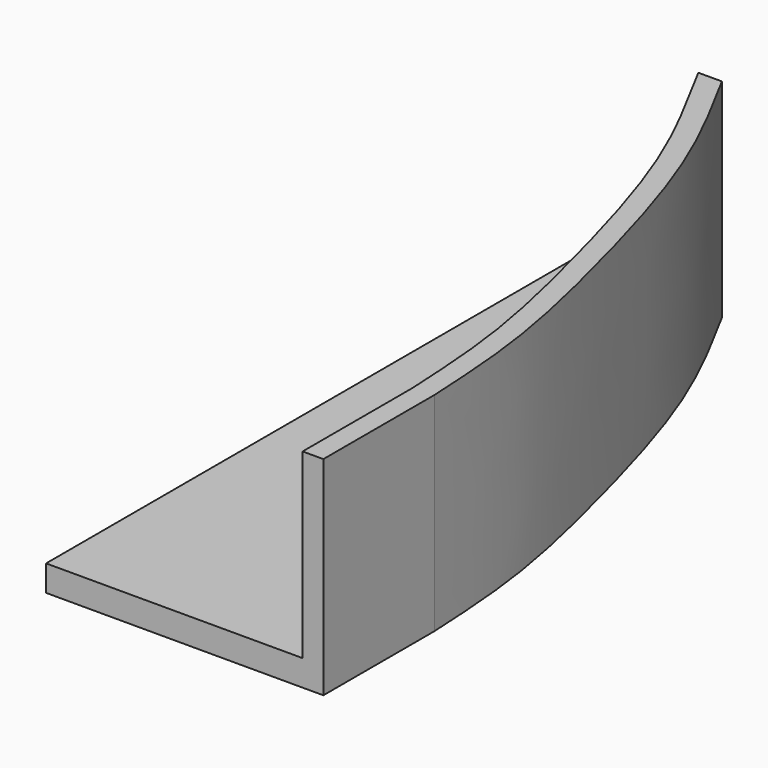
from build123d import *

# Parameters (mm, degrees)
F1_DEPTH = 60
F2_DEPTH = 7.5


# Not quite as in the source:
# - the dataset's text gives a spline's control points without its knots; the knots are read off the source's solid


with BuildPart() as f1:
    # F0 (on Top) → F1 (new body)
    with BuildSketch(Plane.XY):
        with BuildLine():
            Line((-3.4322376549, 127.3491138778), (-10.2491527796, 127.3491138778))
            Line((-10.2491527796, 127.3491138778), (-8.701252002, 124.4790114736))
            add(Edge.make_bspline(
                [(-8.701252002, 124.4790114736), (-7.1362237136, 121.6058887261), (-4.800992375, 117.3185625984), (-1.747416122, 111.541576422), (0.5046891705, 107.1516705554), (2.7109302282, 102.6774335337), (4.5050186798, 98.8556741617), (5.9099551663, 95.7283837822), (6.947576742, 93.3444650289), (7.7980975394, 91.3228569804), (8.4695499974, 89.6828524521), (9.1348820035, 88.0269081744), (9.957166215, 85.9221359954), (11.251973665, 82.4881889813), (12.831222258, 78.0823686514), (14.662666653, 72.6512882748), (16.4302898701, 67.1126017724), (18.134279165, 61.5024770299), (19.7751169491, 55.8567117619), (21.0904401972, 51.1517886054), (22.1119013069, 47.4054001661), (22.8627437246, 44.6087322937), (23.5983740983, 41.8296630381), (24.5595560319, 38.152939528), (25.7198359711, 33.6303684872), (27.0381614496, 28.3164099437), (28.2747953137, 23.1133958726), (29.4220535656, 18.0186567898), (30.4723828119, 13.0297011115), (31.2606871801, 8.9582973415), (31.8355062448, 5.7515670621), (32.2378190146, 3.3713838737), (32.5483276312, 1.4084100397), (32.7814771963, -0.1499496395), (33.0042095884, -1.6999194073), (33.2639776094, -3.6272829064), (33.5480887505, -5.9256145197), (33.806687748, -8.2111304942), (34.1203062464, -11.2436070922), (34.4591587016, -15.0104238238), (34.7976724691, -19.5054666923), (35.1809644079, -25.4820365724), (35.4176012213, -29.9639189701), (35.5761012306, -32.9671092858)],
                knots=[0, 0, 0, 0, 0.0625, 0.09375, 0.125, 0.15625, 0.1875, 0.203125, 0.21875, 0.234375, 0.2421875, 0.25, 0.265625, 0.28125, 0.3125, 0.34375, 0.375, 0.40625, 0.4375, 0.46875, 0.484375, 0.5, 0.515625, 0.53125, 0.5625, 0.59375, 0.625, 0.65625, 0.6875, 0.71875, 0.734375, 0.75, 0.765625, 0.7734375, 0.78125, 0.796875, 0.8125, 0.828125, 0.84375, 0.875, 0.90625, 0.9375, 1, 1, 1, 1], degree=3))
            Line((35.5761012306, -32.9671092858), (35.5761012306, -72.6508861222))
            Line((35.5761012306, -72.6508861222), (41.5677623451, -72.6508861222))
            Line((41.5677623451, -72.6508861222), (41.5677623451, -32.6508861222))
            add(Edge.make_bspline(
                [(-3.4322376549, 127.3491138778), (2.7057866735, 116.0807569713), (15.8535559025, 91.943714127), (30.1753131948, 41.9800249332), (39.8006878737, 0.8308844005), (41.0051328293, -21.9904229426), (41.5677623451, -32.6508861222)],
                knots=[0, 0, 0, 0, 0.2451243363, 0.5250611653, 0.7781429484, 1, 1, 1, 1], degree=3))
        make_face()
    extrude(amount=F1_DEPTH)

    # F0 (on Top) → F2 (join)
    with BuildSketch(Plane.XY):
        with BuildLine():
            Line((-10.2491527796, 127.3491138778), (-38.4322376549, 127.3491138778))
            Line((-38.4322376549, 127.3491138778), (-38.4322376549, -72.6508861222))
            Line((-38.4322376549, -72.6508861222), (35.5761012306, -72.6508861222))
            Line((35.5761012306, -72.6508861222), (35.5761012306, -32.9671092858))
            add(Edge.make_bspline(
                [(-8.701252002, 124.4790114736), (-7.1362237136, 121.6058887261), (-4.800992375, 117.3185625984), (-1.747416122, 111.541576422), (0.5046891705, 107.1516705554), (2.7109302282, 102.6774335337), (4.5050186798, 98.8556741617), (5.9099551663, 95.7283837822), (6.947576742, 93.3444650289), (7.7980975394, 91.3228569804), (8.4695499974, 89.6828524521), (9.1348820035, 88.0269081744), (9.957166215, 85.9221359954), (11.251973665, 82.4881889813), (12.831222258, 78.0823686514), (14.662666653, 72.6512882748), (16.4302898701, 67.1126017724), (18.134279165, 61.5024770299), (19.7751169491, 55.8567117619), (21.0904401972, 51.1517886054), (22.1119013069, 47.4054001661), (22.8627437246, 44.6087322937), (23.5983740983, 41.8296630381), (24.5595560319, 38.152939528), (25.7198359711, 33.6303684872), (27.0381614496, 28.3164099437), (28.2747953137, 23.1133958726), (29.4220535656, 18.0186567898), (30.4723828119, 13.0297011115), (31.2606871801, 8.9582973415), (31.8355062448, 5.7515670621), (32.2378190146, 3.3713838737), (32.5483276312, 1.4084100397), (32.7814771963, -0.1499496395), (33.0042095884, -1.6999194073), (33.2639776094, -3.6272829064), (33.5480887505, -5.9256145197), (33.806687748, -8.2111304942), (34.1203062464, -11.2436070922), (34.4591587016, -15.0104238238), (34.7976724691, -19.5054666923), (35.1809644079, -25.4820365724), (35.4176012213, -29.9639189701), (35.5761012306, -32.9671092858)],
                knots=[0, 0, 0, 0, 0.0625, 0.09375, 0.125, 0.15625, 0.1875, 0.203125, 0.21875, 0.234375, 0.2421875, 0.25, 0.265625, 0.28125, 0.3125, 0.34375, 0.375, 0.40625, 0.4375, 0.46875, 0.484375, 0.5, 0.515625, 0.53125, 0.5625, 0.59375, 0.625, 0.65625, 0.6875, 0.71875, 0.734375, 0.75, 0.765625, 0.7734375, 0.78125, 0.796875, 0.8125, 0.828125, 0.84375, 0.875, 0.90625, 0.9375, 1, 1, 1, 1], degree=3))
            Line((-8.701252002, 124.4790114736), (-10.2491527796, 127.3491138778))
        make_face()
    extrude(amount=F2_DEPTH)


solid = f1.part
